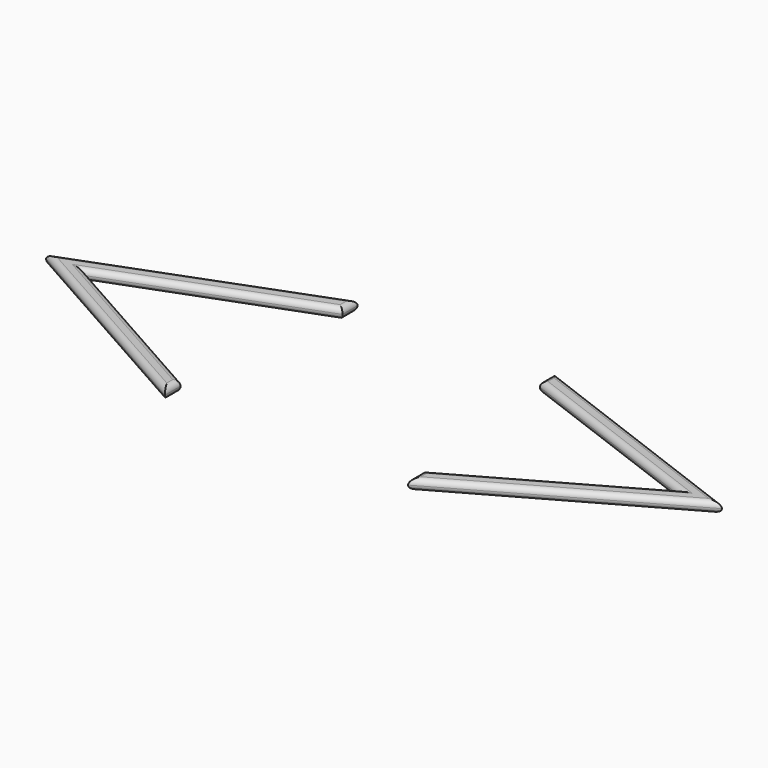
from build123d import *

# Parameters (mm, degrees)
F1_DEPTH = 20
F2_R     = 9.99999


# Not quite as in the source:
# - a fillet or chamfer is up to 0.001 mm smaller than in the source, because OpenCascade refuses the exact size


with BuildPart() as f1:
    # F0 (on Top) → F1 (new body)
    with BuildSketch(Plane.XY):
        Polygon((635.0417733192, 1682.4778318405), (185.4069307446, 1852.2594436146), (185.4069307446, 1816.7974487804), (558.8195690923, 1676.4687693616), (228.5373434424, 1490.2386204266), (228.5373434424, 1453.2696739696), align=None)
    extrude(amount=F1_DEPTH)

    # F2 (radius 10 in the source; OpenCascade refuses exactly that, so slightly less here)
    f2_edges = [f1.edges().sort_by_distance(p)[0] for p in [
        (431.789558, 1567.873753, 20),
        (410.224352, 1767.368638, 20),
        (185.406931, 1834.528446, 20),
        (372.11325, 1746.633109, 20),
        (393.678456, 1583.353695, 20),
        (228.537343, 1471.754147, 20),
        (431.789558, 1567.873753, 0),
        (410.224352, 1767.368638, 0),
        (185.406931, 1834.528446, 0),
        (372.11325, 1746.633109, 0),
        (393.678456, 1583.353695, 0),
        (228.537343, 1471.754147, 0),
    ]]
    fillet(f2_edges, radius=F2_R)


with BuildPart() as f3_1:
    # F3: instance of F1
    add(f1.part.mirror(Plane.YZ))


solid = Compound([f1.part, f3_1.part])
